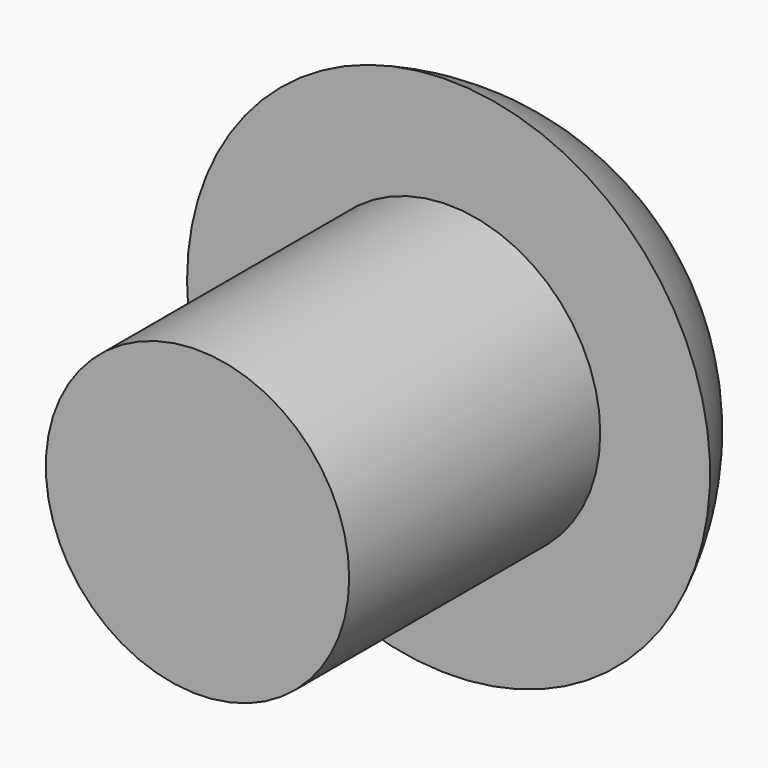
from build123d import *

# Parameters (mm, degrees)
F2_R     = 1.45
F3_DEPTH = 3


# Not quite as in the source:
# - a feature names something its author has since deleted; it is built from what else it names


with BuildPart() as f1:
    # F0 (on Top) → F1 (revolve)
    with BuildSketch(Plane.XY):
        with BuildLine():
            Line((-2.5, 0), (0, 0))
            Line((0, 0), (0, 1.6239797505))
            ThreePointArc((0, 1.6239797505), (-1.4912702214, 1.1834080247), (-2.5, 0))
        make_face()
    revolve(axis=Axis((0, 0.8119898753, 0), (0, 1, 0)))

    # F2 (on face) → F3 (join)
    with BuildSketch(Plane.XZ):
        Circle(F2_R)
    extrude(amount=F3_DEPTH)


solid = f1.part
